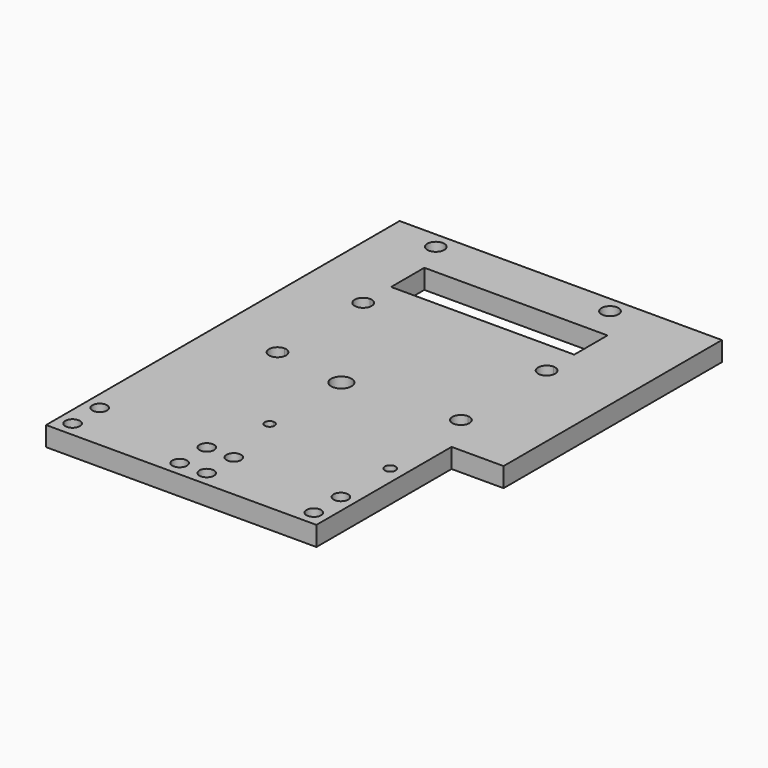
from build123d import *

# Parameters (mm, degrees)
F1_DEPTH  = 4.7625
F2_W      = 23.6109700747
F2_H      = 10.16
F2_W_2    = 21.1328
F3_DEPTH  = 25.4
F4_R      = 2.5
F5_DEPTH  = 25.4
F6_R      = 1.3330740387
F7_DEPTH  = 25.4
F2_R      = 2.0828
F8_DEPTH  = 25.4
F10_DEPTH = 25.4


# Not quite as in the source:
# - a feature names something its author has since deleted; it is built from what else it names


with BuildPart() as f1:
    # F0 (on Top) → F1 (new body)
    with BuildSketch(Plane.XY):
        Polygon((45.72, 53.975), (33.02, 53.975), (-33.02, 53.975), (-33.02, -53.975), (33.02, -53.975), (33.02, -12.7), (45.72, -12.7), align=None)
    extrude(amount=F1_DEPTH)

    # F2 (on face) → F3 (cut)
    with BuildSketch(Plane.XY.offset(4.7625)):
        with Locations((-5.4554850374, 36.7538)):
            Rectangle(F2_W, F2_H)
        with Locations((16.9164, 36.7538)):
            Rectangle(F2_W_2, F2_H)
        with BuildLine():
            ThreePointArc((29.5656, 23.241), (28.9555620039, 24.7137620039), (27.4828, 25.3238))
            Line((27.4828, 25.3238), (27.4828, 21.1582))
            ThreePointArc((27.4828, 21.1582), (28.9555620039, 21.7682379961), (29.5656, 23.241))
        make_face()
        with BuildLine():
            Line((27.4828, 21.1582), (27.4828, 25.3238))
            ThreePointArc((27.4828, 25.3238), (25.4, 23.241), (27.4828, 21.1582))
        make_face()
        with BuildLine():
            ThreePointArc((27.4828, -0.8382), (25.4, -2.921), (27.4828, -5.0038))
            Line((27.4828, -5.0038), (27.4828, -0.8382))
        make_face()
        with BuildLine():
            Line((27.4828, -0.8382), (27.4828, -5.0038))
            ThreePointArc((27.4828, -5.0038), (28.9555620039, -4.3937620039), (29.5656, -2.921))
            ThreePointArc((29.5656, -2.921), (28.9555620039, -1.4482379961), (27.4828, -0.8382))
        make_face()
        with BuildLine():
            ThreePointArc((-15.24, 23.241), (-15.8500379961, 24.7137620039), (-17.3228, 25.3238))
            Line((-17.3228, 25.3238), (-17.3228, 21.1582))
            ThreePointArc((-17.3228, 21.1582), (-15.8500379961, 21.7682379961), (-15.24, 23.241))
        make_face()
        with BuildLine():
            Line((-17.3228, 21.1582), (-17.3228, 25.3238))
            ThreePointArc((-17.3228, 25.3238), (-19.4056, 23.241), (-17.3228, 21.1582))
        make_face()
        with BuildLine():
            ThreePointArc((-17.3228, -0.8382), (-19.4056, -2.921), (-17.3228, -5.0038))
            Line((-17.3228, -5.0038), (-17.3228, -0.8382))
        make_face()
        with BuildLine():
            Line((-17.3228, -0.8382), (-17.3228, -5.0038))
            ThreePointArc((-17.3228, -5.0038), (-15.8500379961, -4.3937620039), (-15.24, -2.921))
            ThreePointArc((-15.24, -2.921), (-15.8500379961, -1.4482379961), (-17.3228, -0.8382))
        make_face()
    extrude(amount=-F3_DEPTH, mode=Mode.SUBTRACT)

    # F4 (on face) → F5 (cut)
    with BuildSketch(Plane(origin=(0, 0, 0), x_dir=(1, 0, 0), z_dir=(0, 0, -1))):
        with Locations((0, 5.08)):
            Circle(F4_R)
    extrude(amount=-F5_DEPTH, mode=Mode.SUBTRACT)

    # F6 (on face) → F7 (cut)
    with BuildSketch(Plane.XY.offset(4.7625)):
        with BuildLine():
            Line((0, -28.178125), (0, -25.796875))
            ThreePointArc((0, -25.796875), (-1.190625, -26.9875), (0, -28.178125))
        make_face()
        with BuildLine():
            ThreePointArc((0, -28.178125), (0.8418990114, -27.8293990114), (1.190625, -26.9875))
            ThreePointArc((1.190625, -26.9875), (0.8418990114, -26.1456009886), (0, -25.796875))
            Line((0, -25.796875), (0, -28.178125))
        make_face()
        with Locations((29.460657388, -26.9875)):
            Circle(F6_R)
    extrude(amount=-F7_DEPTH, mode=Mode.SUBTRACT)

    # F2 (on face) → F8 (cut)
    with BuildSketch(Plane.XY.offset(4.7625)):
        with Locations((-20.9680330008, 49.9618)):
            Circle(F2_R)
        with BuildLine():
            ThreePointArc((23.6728, 49.9618), (21.59, 52.0446), (19.5072, 49.9618))
            ThreePointArc((19.5072, 49.9618), (21.59, 47.879), (23.6728, 49.9618))
        make_face()
    extrude(amount=-F8_DEPTH, mode=Mode.SUBTRACT)

    # F9 (on face) → F10 (cut)
    with BuildSketch(Plane.XY.offset(4.7625)):
        with BuildLine():
            Line((-29.464, -48.5479413316), (-29.464, -52.1039413316))
            ThreePointArc((-29.464, -52.1039413316), (-28.2067641431, -51.5831771885), (-27.686, -50.3259413316))
            ThreePointArc((-27.686, -50.3259413316), (-28.2067641431, -49.0687054746), (-29.464, -48.5479413316))
        make_face()
        with BuildLine():
            ThreePointArc((-29.464, -48.5479413316), (-31.242, -50.3259413316), (-29.464, -52.1039413316))
            Line((-29.464, -52.1039413316), (-29.464, -48.5479413316))
        make_face()
        with BuildLine():
            ThreePointArc((-27.686, -42.0469199679), (-28.2067641431, -40.7896841109), (-29.464, -40.2689199679))
            Line((-29.464, -40.2689199679), (-29.464, -43.8249199679))
            ThreePointArc((-29.464, -43.8249199679), (-28.2067641431, -43.3041558248), (-27.686, -42.0469199679))
        make_face()
        with BuildLine():
            Line((-29.464, -43.8249199679), (-29.464, -40.2689199679))
            ThreePointArc((-29.464, -40.2689199679), (-31.242, -42.0469199679), (-29.464, -43.8249199679))
        make_face()
        with BuildLine():
            Line((-3.302, -43.8249199679), (-3.302, -40.2689199679))
            ThreePointArc((-3.302, -40.2689199679), (-5.08, -42.0469199679), (-3.302, -43.8249199679))
        make_face()
        with BuildLine():
            ThreePointArc((-1.524, -42.0469199679), (-2.0447641431, -40.7896841109), (-3.302, -40.2689199679))
            Line((-3.302, -40.2689199679), (-3.302, -43.8249199679))
            ThreePointArc((-3.302, -43.8249199679), (-2.0447641431, -43.3041558248), (-1.524, -42.0469199679))
        make_face()
        with BuildLine():
            ThreePointArc((-3.302, -48.5479413316), (-5.08, -50.3259413316), (-3.302, -52.1039413316))
            Line((-3.302, -52.1039413316), (-3.302, -48.5479413316))
        make_face()
        with BuildLine():
            Line((-3.302, -48.5479413316), (-3.302, -52.1039413316))
            ThreePointArc((-3.302, -52.1039413316), (-2.0447641431, -51.5831771885), (-1.524, -50.3259413316))
            ThreePointArc((-1.524, -50.3259413316), (-2.0447641431, -49.0687054746), (-3.302, -48.5479413316))
        make_face()
        with BuildLine():
            ThreePointArc((3.302, -48.5479413316), (1.524, -50.3259413316), (3.302, -52.1039413316))
            Line((3.302, -52.1039413316), (3.302, -48.5479413316))
        make_face()
        with BuildLine():
            Line((3.302, -48.5479413316), (3.302, -52.1039413316))
            ThreePointArc((3.302, -52.1039413316), (4.5592358569, -51.5831771885), (5.08, -50.3259413316))
            ThreePointArc((5.08, -50.3259413316), (4.5592358569, -49.0687054746), (3.302, -48.5479413316))
        make_face()
        with BuildLine():
            ThreePointArc((5.08, -42.0469199679), (4.5592358569, -40.7896841109), (3.302, -40.2689199679))
            Line((3.302, -40.2689199679), (3.302, -43.8249199679))
            ThreePointArc((3.302, -43.8249199679), (4.5592358569, -43.3041558248), (5.08, -42.0469199679))
        make_face()
        with BuildLine():
            Line((3.302, -43.8249199679), (3.302, -40.2689199679))
            ThreePointArc((3.302, -40.2689199679), (1.524, -42.0469199679), (3.302, -43.8249199679))
        make_face()
        with BuildLine():
            Line((29.464, -43.8249199679), (29.464, -40.2689199679))
            ThreePointArc((29.464, -40.2689199679), (27.686, -42.0469199679), (29.464, -43.8249199679))
        make_face()
        with BuildLine():
            ThreePointArc((31.242, -42.0469199679), (30.7212358569, -40.7896841109), (29.464, -40.2689199679))
            Line((29.464, -40.2689199679), (29.464, -43.8249199679))
            ThreePointArc((29.464, -43.8249199679), (30.7212358569, -43.3041558248), (31.242, -42.0469199679))
        make_face()
        with BuildLine():
            Line((29.464, -48.5479413316), (29.464, -52.1039413316))
            ThreePointArc((29.464, -52.1039413316), (30.7212358569, -51.5831771885), (31.242, -50.3259413316))
            ThreePointArc((31.242, -50.3259413316), (30.7212358569, -49.0687054746), (29.464, -48.5479413316))
        make_face()
        with BuildLine():
            ThreePointArc((29.464, -48.5479413316), (27.686, -50.3259413316), (29.464, -52.1039413316))
            Line((29.464, -52.1039413316), (29.464, -48.5479413316))
        make_face()
    extrude(amount=-F10_DEPTH, mode=Mode.SUBTRACT)


solid = f1.part
